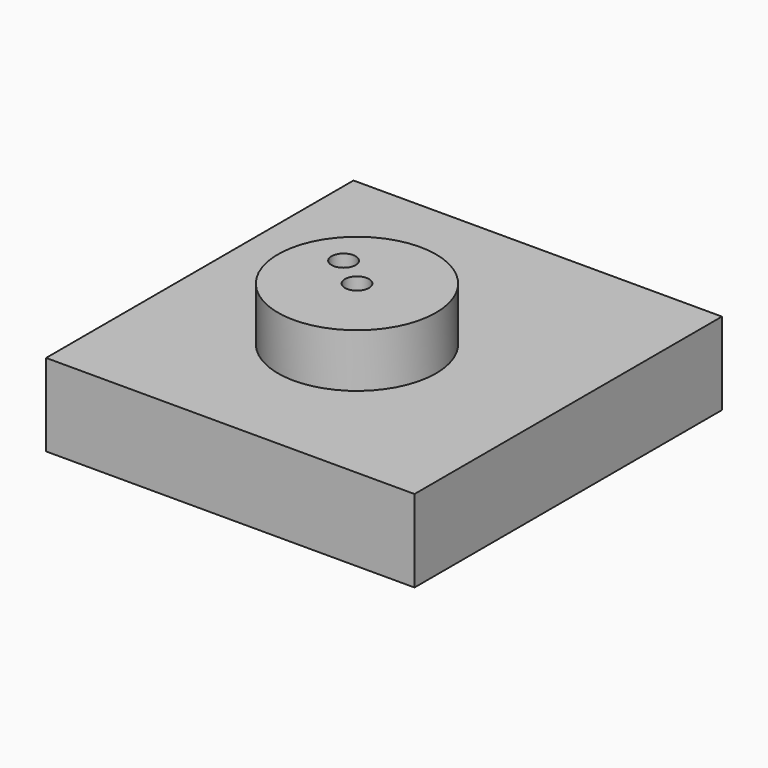
from build123d import *

# Parameters (mm, degrees)
F1_DEPTH   = 21.6836184263
F2_R       = 20.8194643485
F3_DEPTH   = 14.0719488263
F7_D       = 6.35
F7_DEPTH   = 14.0729488263
F7_ON_F6_D = 6.35


# Not quite as in the source:
# - the program builds the solid bodies; features that only make, move or delete a surface that nothing else refers to are left out


with BuildPart() as f1:
    # F0 (on Top) → F1 (new body)
    with BuildSketch(Plane.XY):
        Polygon((50.926592201, 50.2595603466), (-46.1172051728, 50.2595603466), (-46.1172051728, -50.9577989578), (50.926592201, -50.9577989578), (50.926592201, 48.6862957478), align=None)
    extrude(amount=F1_DEPTH)

    # F2 (on face) → F3 (join)
    with BuildSketch(Plane.XY.offset(21.6836184263)):
        with Locations((0, -6.2367771752)):
            Circle(F2_R)
    extrude(amount=F3_DEPTH)

    # F7 (through all, one way)
    with BuildSketch(Plane(origin=(0, 0, 21.6836184263), x_dir=(1, 0, 0), z_dir=(0, 0, -1))):
        with Locations((0, 6.2367771752)):
            Circle(F7_D / 2)
    extrude(amount=-F7_DEPTH, mode=Mode.SUBTRACT)

    # F7 on F6 (through all)
    with Locations(Plane(origin=(0, 0, 0), x_dir=(1, 0, 0), z_dir=(0, 0, -1))):
        with Locations((-8.5173435509, 0)):
            Hole(F7_ON_F6_D / 2)


solid = f1.part
